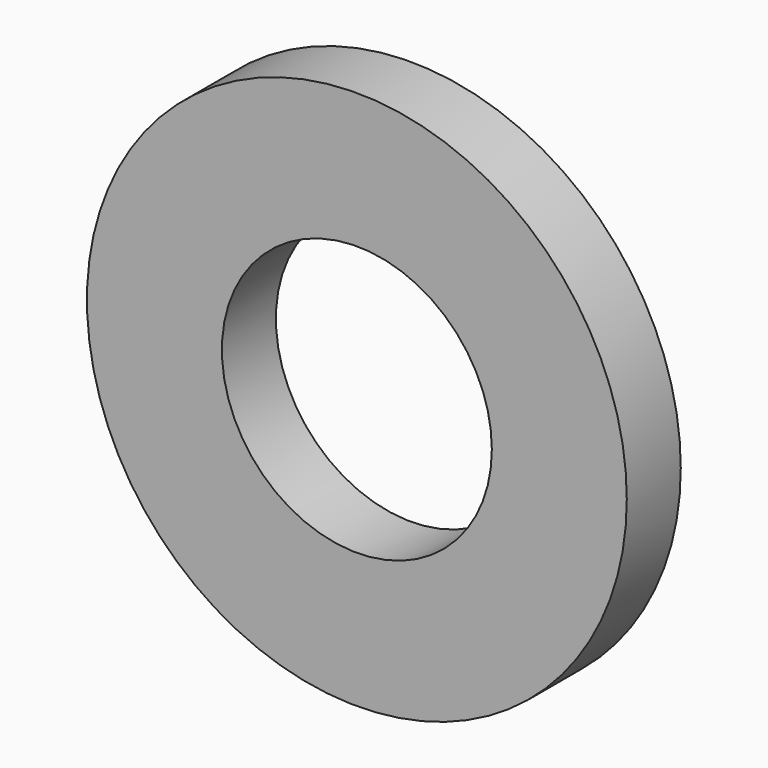
from build123d import *

# Parameters (mm, degrees)
F1_R     = 12.7
F1_R_2   = 6.35
F2_DEPTH = 3.175


with BuildPart() as f2:
    # F1 (on Front) → F2 (new body)
    with BuildSketch(Plane.XZ):
        Circle(F1_R)
        Circle(F1_R_2, mode=Mode.SUBTRACT)
    extrude(amount=F2_DEPTH)


solid = f2.part
